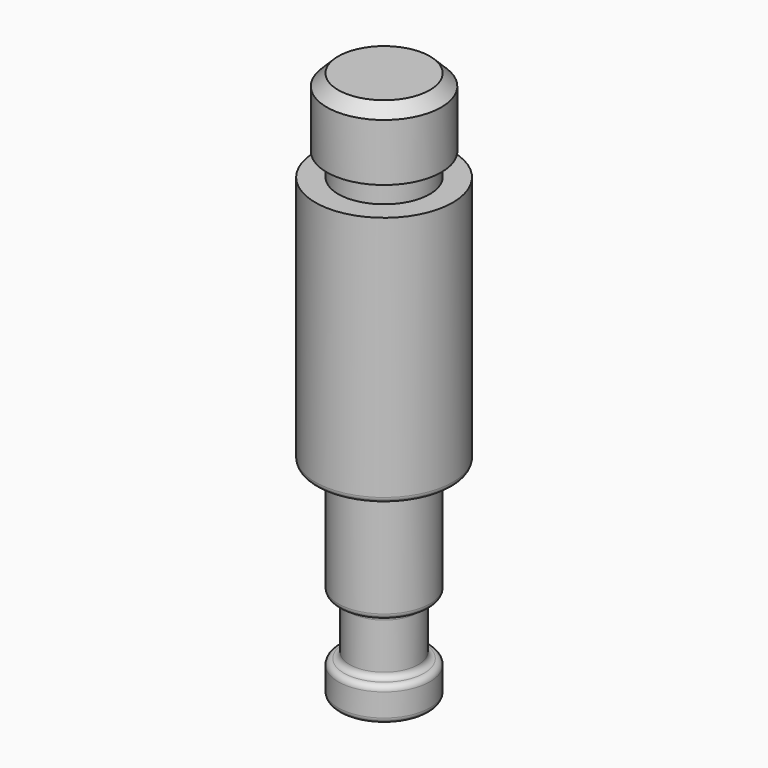
from build123d import *

# Parameters (mm, degrees)
F0_R     = 6
F1_DEPTH = 40
F2_R     = 5
F3_DEPTH = 8
F6_R     = 0.49999
F7_W     = 1
F7_H     = 2
F9_SIZE  = 1


# Not quite as in the source:
# - a fillet or chamfer is up to 0.001 mm smaller than in the source, because OpenCascade refuses the exact size


with BuildPart() as f1:
    # F0 (on Top) → F1 (new body)
    with BuildSketch(Plane.XY):
        Circle(F0_R)
    extrude(amount=-F1_DEPTH)

    # F2 (on face) → F3 (join)
    with BuildSketch(Plane.XY):
        Circle(F2_R)
    extrude(amount=F3_DEPTH)

    # F4 (on Right) → F5 (revolve, cut)
    with BuildSketch(Plane.YZ):
        Polygon((-6, -22), (-6, -40), (-4, -40), (-4, -37), (-3, -37), (-3, -32), (-4, -32), (-4, -22), align=None)
    revolve(axis=Axis((0, 0, -26.2926705182), (0, 0, 1)), mode=Mode.SUBTRACT)

    # F6 (radius 0.5 in the source; OpenCascade refuses exactly that, so slightly less here)
    f6_edges = [f1.edges().sort_by_distance(p)[0] for p in [
        (0, 4, -40),
        (0, 4, -37),
        (0, 3, -37),
        (0, 3, -32),
        (0, 4, -32),
        (0, 4, -22),
        (-6, 0, -22),
    ]]
    fillet(f6_edges, radius=F6_R)

    # F7 (on Right) → F8 (revolve, cut)
    with BuildSketch(Plane.YZ):
        with Locations((-4.5, 1)):
            Rectangle(F7_W, F7_H)
    revolve(axis=Axis((0, 0, 11.1455004662), (0, 0, 1)), mode=Mode.SUBTRACT)

    # F9
    f9_edges = [f1.edges().sort_by_distance(p)[0] for p in [
        (-5, 0, 8),
    ]]
    chamfer(f9_edges, length=F9_SIZE)


solid = f1.part
